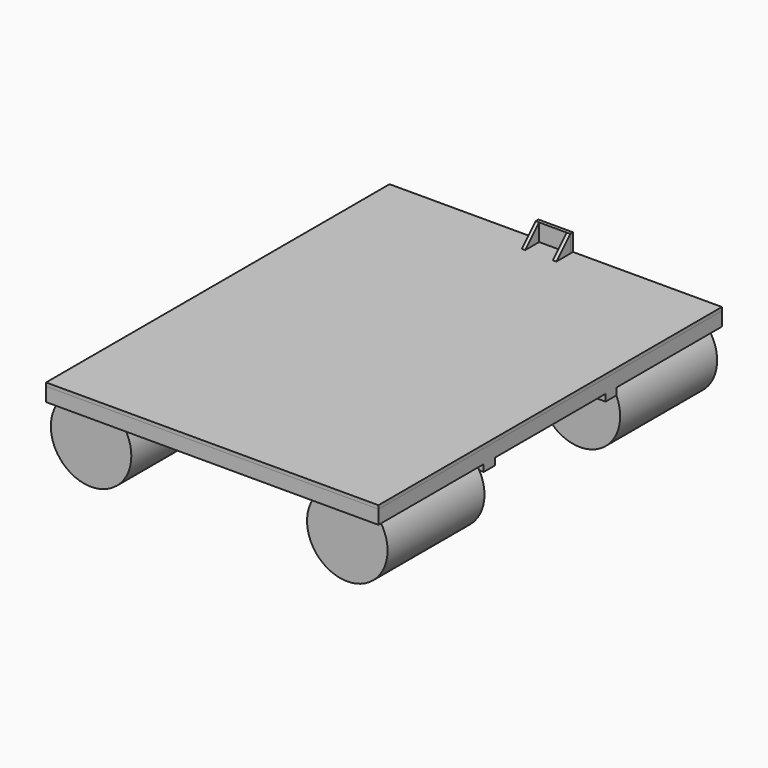
from build123d import *

# Parameters (mm, degrees)
F0_W      = 50.8
F0_H      = 3048
F1_DEPTH  = 101.6
F6_W      = 101.6
F6_H      = 50.8
F7_DEPTH  = 2438.4
F5_R      = 295.275
F8_DEPTH  = 889
F9_R      = 295.275
F10_DEPTH = 889
F12_W     = 127
F12_H     = 25.4
F13_DEPTH = 25.4
F14_DEPTH = 152.4
F16_DEPTH = 25.4
F18_DEPTH = 25.4


with BuildPart() as f1:
    # F0 (on Top) → F1 (new body)
    with BuildSketch(Plane.XY):
        Polygon((-2145.970582962, 2768.0247317466), (-2145.970582962, 2717.2247317466), (-2095.170582962, 2717.2247317466), (-1637.970582962, 2717.2247317466), (-1587.170582962, 2717.2247317466), (-1079.170582962, 2717.2247317466), (-1028.370582962, 2717.2247317466), (-825.170582962, 2717.2247317466), (-774.370582962, 2717.2247317466), (-266.370582962, 2717.2247317466), (-215.570582962, 2717.2247317466), (241.629417038, 2717.2247317466), (292.429417038, 2717.2247317466), (292.429417038, 2768.0247317466), align=None)
        with Locations((-2120.570582962, 1193.2247317466)):
            Rectangle(F0_W, F0_H)
        Polygon((-2095.170582962, -330.7752682534), (-2145.970582962, -330.7752682534), (-2145.970582962, -381.5752682534), (292.429417038, -381.5752682534), (292.429417038, -330.7752682534), (241.629417038, -330.7752682534), (-215.570582962, -330.7752682534), (-266.370582962, -330.7752682534), (-774.370582962, -330.7752682534), (-825.170582962, -330.7752682534), (-1028.370582962, -330.7752682534), (-1079.170582962, -330.7752682534), (-1587.170582962, -330.7752682534), (-1637.970582962, -330.7752682534), align=None)
        with Locations((267.029417038, 1193.2247317466)):
            Rectangle(F0_W, F0_H)
        with Locations((-1612.570582962, 1193.2247317466)):
            Rectangle(F0_W, F0_H)
        with Locations((-1053.770582962, 1193.2247317466)):
            Rectangle(F0_W, F0_H)
        with Locations((-799.770582962, 1193.2247317466)):
            Rectangle(F0_W, F0_H)
        with Locations((-240.970582962, 1193.2247317466)):
            Rectangle(F0_W, F0_H)
    extrude(amount=F1_DEPTH)

    # F6 (on offset) → F7 (join)
    with BuildSketch(Plane(origin=(292.429417038, 0, 0), x_dir=(0, -1, 0), z_dir=(-1, 0, 0))):
        with Locations((-634.4247317466, -25.4)):
            Rectangle(F6_W, F6_H)
        with Locations((-1752.0247317466, -25.4)):
            Rectangle(F6_W, F6_H)
    extrude(amount=F7_DEPTH)


with BuildPart() as f8:
    # F5 (on offset) → F8 (new body)
    with BuildSketch(Plane.XZ.offset(318.0752682534)):
        with Locations((13.029417038, -186.8939956901)):
            Circle(F5_R)
    extrude(amount=-F8_DEPTH)


with BuildPart() as f8b:
    # F5 (on offset) → F8, piece 2 (new body)
    with BuildSketch(Plane.XZ.offset(318.0752682534)):
        with Locations((-1866.570582962, -186.8939956901)):
            Circle(F5_R)
    extrude(amount=-F8_DEPTH)


with BuildPart() as f10:
    # F9 (on offset) → F10 (new body)
    with BuildSketch(Plane(origin=(0, 2704.5247317466, 0), x_dir=(-1, 0, 0), z_dir=(0, 1, 0))):
        with Locations((-13.029417038, -186.8939956901)):
            Circle(F9_R)
    extrude(amount=-F10_DEPTH)


with BuildPart() as f10b:
    # F9 (on offset) → F10, piece 2 (new body)
    with BuildSketch(Plane(origin=(0, 2704.5247317466, 0), x_dir=(-1, 0, 0), z_dir=(0, 1, 0))):
        with Locations((1866.570582962, -186.8939956901)):
            Circle(F9_R)
    extrude(amount=-F10_DEPTH)


with BuildPart() as f13:
    # F12 (on offset) → F13 (new body)
    with BuildSketch(Plane.XY.offset(101.6)):
        Polygon((-1053.770582962, 2768.0247317466), (-2145.970582962, 2768.0247317466), (-2145.970582962, -381.5752682534), (-926.770582962, -381.5752682534), (-926.770582962, 2742.6247317466), (-1053.770582962, 2742.6247317466), align=None)
        Polygon((-1028.370582962, 2768.0247317466), (-1053.770582962, 2768.0247317466), (-1053.770582962, 2742.6247317466), (-926.770582962, 2742.6247317466), (-926.770582962, 2768.0247317466), align=None)
        Polygon((-926.770582962, 2742.6247317466), (-926.770582962, -381.5752682534), (292.429417038, -381.5752682534), (292.429417038, 2768.0247317466), (-799.770582962, 2768.0247317466), (-799.770582962, 2742.6247317466), align=None)
        with Locations((-863.270582962, 2755.3247317466)):
            Rectangle(F12_W, F12_H)
    extrude(amount=F13_DEPTH)

    # F15 (on face) → F16 (join)
    with BuildSketch(Plane.YZ.offset(-799.770582962)):
        Polygon((2742.6247317466, 127), (2742.6247317466, 254), (2615.6247317466, 127), align=None)
    extrude(amount=-F16_DEPTH)

    # F17 (on face) → F18 (join)
    with BuildSketch(Plane(origin=(-1053.770582962, 0, 0), x_dir=(0, -1, 0), z_dir=(-1, 0, 0))):
        Polygon((-2742.6247317466, 127), (-2615.6247317466, 127), (-2742.6247317466, 254), align=None)
    extrude(amount=-F18_DEPTH)


with BuildPart() as f14:
    # F12 (on offset) → F14 (new body)
    with BuildSketch(Plane.XY.offset(101.6)):
        Polygon((-1028.370582962, 2768.0247317466), (-1053.770582962, 2768.0247317466), (-1053.770582962, 2742.6247317466), (-926.770582962, 2742.6247317466), (-926.770582962, 2768.0247317466), align=None)
        with Locations((-863.270582962, 2755.3247317466)):
            Rectangle(F12_W, F12_H)
    extrude(amount=F14_DEPTH)


solid = Compound([f1.part, f8.part, f8b.part, f10.part, f10b.part, f13.part, f14.part])
